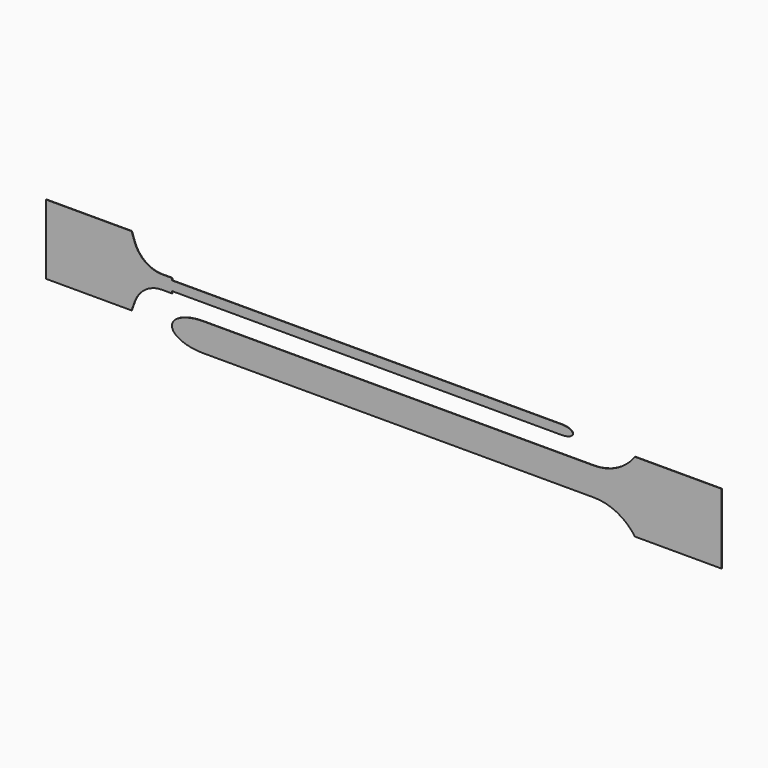
from build123d import *

# Parameters (mm, degrees)
F2_DEPTH = 0.0508


# Not quite as in the source:
# - ends of sketch curves that miss each other by under 0.0002 mm in the source are joined


with BuildPart() as f2:
    # F0 (on Front) → F2 (new body)
    with BuildSketch(Plane.XZ):
        with BuildLine():
            Line((-22.2519018109, 2.7154037545), (-31.5314531326, 2.7154037545))
            Line((-31.5314531326, 2.7154037545), (-31.5314531326, -4.8547233455))
            Line((-31.5314531326, -4.8547233455), (-22.2519018109, -4.8547233455))
            Line((-22.2519018109, -4.8547233455), (-21.9214119342, -3.9214320238))
            ThreePointArc((-21.9214119342, -3.9214320238), (-20.7609625105, -2.3884201716), (-18.9285192327, -1.8062519505))
            Line((-18.9285192327, -1.8062519505), (-17.8517878327, -1.8062519505))
            Line((-17.8517878327, -1.8062519505), (-17.8517878327, -1.577656713))
            Line((-17.8517878327, -1.577656713), (24.3993468673, -1.577656713))
            add(Edge.make_bspline(
                [(24.3993468673, -1.577656713), (25.6243397865, -1.577656713), (25.6243397865, -1.0696597955), (25.6243397865, -0.5616628779), (24.3993468673, -0.5616628779)],
                knots=[4.7123889804, 4.7123889804, 4.7123889804, 6.2831853072, 6.2831853072, 7.853981634, 7.853981634, 7.853981634], degree=2, weights=[1, 0.7071067812, 1, 0.7071067812, 1]))
            Line((24.3993468673, -0.5616628779), (-17.8517878327, -0.5616628779))
            Line((-17.8517878327, -0.5616628779), (-17.8517878327, -0.3330676404))
            Line((-17.8517878327, -0.3330676404), (-18.9285192327, -0.3330676404))
            ThreePointArc((-18.9285192327, -0.3330676404), (-20.7609625105, 0.2491005807), (-21.9214119342, 1.7821124329))
            Line((-21.9214119342, 1.7821124329), (-22.2519018109, 2.7154037545))
        make_face()
    extrude(amount=F2_DEPTH)


with BuildPart() as f2b:
    # F1 (on Front) → F2, piece 2 (new body)
    with BuildSketch(Plane.XZ):
        with BuildLine():
            Line((27.9137630355, -3.3628604373), (-14.5042369645, -3.3628604373))
            Line((-14.5042369645, -3.3628604373), (-14.9646373645, -3.3770590373))
            Line((-14.9646373645, -3.3770590373), (-15.4164525645, -3.4193754373))
            Line((-15.4164525645, -3.4193754373), (-15.8512751645, -3.4890222373))
            Line((-15.8512751645, -3.4890222373), (-16.2610025645, -3.5847294373))
            Line((-16.2610025645, -3.5847294373), (-16.6380147645, -3.7046682373))
            Line((-16.6380147645, -3.7046682373), (-16.9752759645, -3.8466542373))
            Line((-16.9752759645, -3.8466542373), (-17.2665123645, -4.0079950373))
            Line((-17.2665123645, -4.0079950373), (-17.5062883645, -4.1857188373))
            Line((-17.5062883645, -4.1857188373), (-17.6901335645, -4.3764982373))
            Line((-17.6901335645, -4.3764982373), (-17.8146443645, -4.5768026373))
            Line((-17.8146443645, -4.5768026373), (-17.8774585645, -4.7828474373))
            Line((-17.8774585645, -4.7828474373), (-17.8774585645, -4.9908734373))
            Line((-17.8774585645, -4.9908734373), (-17.8146443645, -5.1969182373))
            Line((-17.8146443645, -5.1969182373), (-17.6901335645, -5.3972226373))
            Line((-17.6901335645, -5.3972226373), (-17.5062883645, -5.5880020373))
            Line((-17.5062883645, -5.5880020373), (-17.2665123645, -5.7657258373))
            Line((-17.2665123645, -5.7657258373), (-16.9752759645, -5.9270666373))
            Line((-16.9752759645, -5.9270666373), (-16.6380147645, -6.0690526373))
            Line((-16.6380147645, -6.0690526373), (-16.2610025645, -6.1889914373))
            Line((-16.2610025645, -6.1889914373), (-15.8512751645, -6.2846986373))
            Line((-15.8512751645, -6.2846986373), (-15.4164525645, -6.3543454373))
            Line((-15.4164525645, -6.3543454373), (-14.9646373645, -6.3966618373))
            Line((-14.9646373645, -6.3966618373), (-14.5042369645, -6.4108604373))
            Line((-14.5042369645, -6.4108604373), (27.9137630355, -6.4108604373))
            ThreePointArc((27.9137630355, -6.4108604373), (30.4129542245, -7.0158501043), (32.3587639958, -8.6968597505))
            Line((32.3587639958, -8.6968597505), (41.7567630355, -8.6968604373))
            Line((41.7567630355, -8.6968604373), (41.7567630355, -1.0768604373))
            Line((41.7567630355, -1.0768604373), (32.3587630355, -1.0768604373))
            ThreePointArc((32.3587630355, -1.0768604373), (30.4129542245, -2.7578707702), (27.9137630355, -3.3628604373))
        make_face()
    extrude(amount=F2_DEPTH)


solid = Compound([f2.part, f2b.part])
